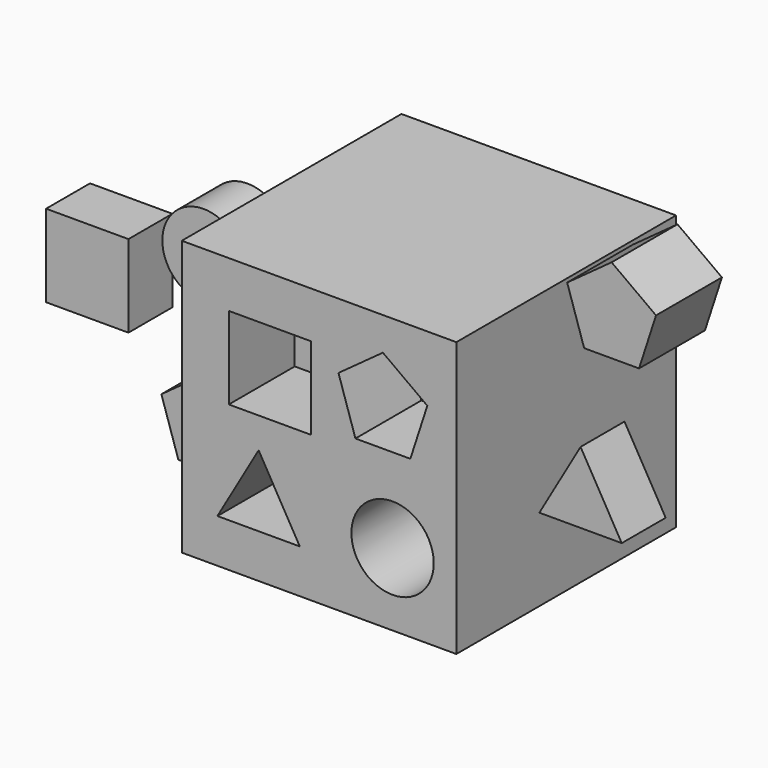
from build123d import *

# Parameters (mm, degrees)
F0_W      = 127
F0_H      = 127
F1_DEPTH  = 63.5
F2_W      = 38.1
F2_H      = 38.1
F3_DEPTH  = 38.1
F5_DEPTH  = 38.1
F6_R      = 19.05
F8_DEPTH  = 38.1
F9_DEPTH  = 38.1
F10_W     = 38.1
F10_H     = 38.1
F11_DEPTH = 25.4
F13_DEPTH = 25.4
F12_R     = 19.05
F14_DEPTH = 25.4
F16_DEPTH = 38.1


# Not quite as in the source:
# - a feature of the source that left no trace in its solid (it failed there, or was rolled back) is left out
# - a feature names something its author has since deleted; it is built from what else it names


with BuildPart() as f1:
    # F0 (on Front) → F1 (new body, symmetric)
    with BuildSketch(Plane.XZ):
        with Locations((1.0360684865, -0.8295979351)):
            Rectangle(F0_W, F0_H)
    extrude(amount=F1_DEPTH, both=True)

    # F2 (on face) → F3 (cut)
    with BuildSketch(Plane.XZ.offset(63.5)):
        with Locations((-21.6616940452, 22.1276779154)):
            Rectangle(F2_W, F2_H)
    extrude(amount=-F3_DEPTH, mode=Mode.SUBTRACT)

    # F4 (on face) → F5 (cut)
    with BuildSketch(Plane.XZ.offset(63.5)):
        Polygon((43.2534851908, 8.2597824623), (51.102516848, 32.4166179762), (30.5534851908, 47.3463633845), (10.0044535337, 32.4166179762), (17.8534851908, 8.2597824623), align=None)
    extrude(amount=-F5_DEPTH, mode=Mode.SUBTRACT)

    # F6 (on face) → F8 (cut)
    with BuildSketch(Plane.XZ.offset(63.5)):
        with Locations((35.0274220109, -30.7872574776)):
            Circle(F6_R)
        Polygon((-26.9323371144, -11.076669144), (-45.9823371144, -44.0722370282), (-7.8823371144, -44.0722370282), align=None)
    extrude(amount=-F8_DEPTH, mode=Mode.SUBTRACT)

    # F6 (on face) → F9 (cut)
    with BuildSketch(Plane.XZ.offset(63.5)):
        with Locations((35.0274220109, -30.7872574776)):
            Circle(F6_R)
        Polygon((-26.9323371144, -11.076669144), (-45.9823371144, -44.0722370282), (-7.8823371144, -44.0722370282), align=None)
    extrude(amount=-F9_DEPTH, mode=Mode.SUBTRACT)


with BuildPart() as f11:
    # F10 (on Front) → F11 (new body)
    with BuildSketch(Plane.XZ):
        with Locations((-136.6716623306, 10.8564948447)):
            Rectangle(F10_W, F10_H)
    extrude(amount=F11_DEPTH)


with BuildPart() as f13:
    # F12 (on Front) → F13 (new body)
    with BuildSketch(Plane.XZ):
        Polygon((-102.3873424113, -28.2908431806), (-94.5383107541, -52.4476786945), (-69.1383107541, -52.4476786945), (-61.289279097, -28.2908431806), (-81.8383107541, -13.3610977723), align=None)
    extrude(amount=F13_DEPTH)


with BuildPart() as f13b:
    # F12 (on Front) → F13, piece 2 (new body)
    with BuildSketch(Plane.XZ):
        with Locations((-82.8998610377, 34.4743542373)):
            Circle(F12_R)
    extrude(amount=F13_DEPTH)


with BuildPart() as f13c:
    # F12 (on Front) → F13, piece 3 (new body)
    with BuildSketch(Plane.XZ):
        Polygon((91.5077158689, 13.3103162459), (72.4577158689, -19.6852516383), (110.5577158689, -19.6852516383), align=None)
    extrude(amount=F13_DEPTH)


with BuildPart() as f14:
    # F12 (on Front) → F14 (new body)
    with BuildSketch(Plane.XZ):
        Polygon((-102.3873424113, -28.2908431806), (-94.5383107541, -52.4476786945), (-69.1383107541, -52.4476786945), (-61.289279097, -28.2908431806), (-81.8383107541, -13.3610977723), align=None)
    extrude(amount=F14_DEPTH)


with BuildPart() as f14b:
    # F12 (on Front) → F14, piece 2 (new body)
    with BuildSketch(Plane.XZ):
        with Locations((-82.8998610377, 34.4743542373)):
            Circle(F12_R)
    extrude(amount=F14_DEPTH)


with BuildPart() as f14c:
    # F12 (on Front) → F14, piece 3 (new body)
    with BuildSketch(Plane.XZ):
        Polygon((91.5077158689, 13.3103162459), (72.4577158689, -19.6852516383), (110.5577158689, -19.6852516383), align=None)
    extrude(amount=F14_DEPTH)


with BuildPart() as f16:
    # F15 (on Front) → F16 (new body)
    with BuildSketch(Plane.XZ):
        Polygon((128.7221174359, 62.5196497987), (136.5711490931, 86.6764853125), (116.0221174359, 101.6062307208), (95.4730857788, 86.6764853125), (103.3221174359, 62.5196497987), align=None)
    extrude(amount=F16_DEPTH)


solid = Compound([f1.part, f11.part, f13.part, f13b.part, f13c.part, f14.part, f14b.part, f14c.part, f16.part])
